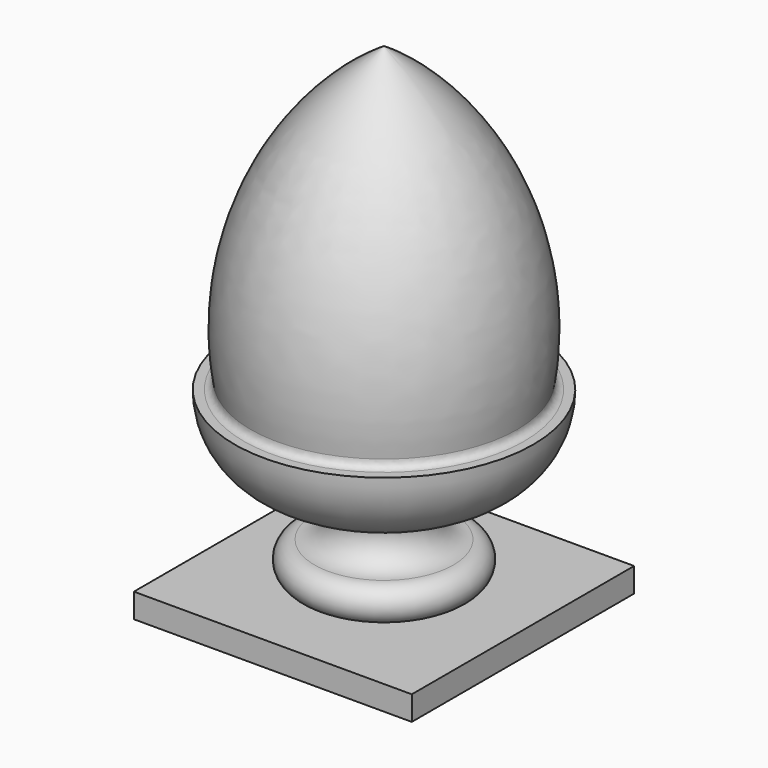
from build123d import *

# Parameters (mm, degrees)
F0_W     = 203.2
F0_H     = 203.2
F1_DEPTH = 17.78
F4_R     = 5.08


# Not quite as in the source:
# - a feature names something its author has since deleted; it is built from what else it names


with BuildPart() as f1:
    # F0 (on Top) → F1 (new body)
    with BuildSketch(Plane.XY):
        Rectangle(F0_W, F0_H)
    extrude(amount=F1_DEPTH)

    # F2 (on Front) → F3 (revolve)
    with BuildSketch(Plane.XZ):
        with BuildLine():
            Line((0, 360.68), (0, 17.78))
            Line((0, 17.78), (50.8, 17.78))
            ThreePointArc((50.8, 17.78), (63.5, 30.48), (50.8, 43.18))
            ThreePointArc((50.8, 43.18), (31.75, 62.23), (50.8, 81.28))
            ThreePointArc((50.8, 81.28), (92.1091781569, 98.3908218431), (109.22, 139.7))
            Line((109.22, 139.7), (96.52, 139.7))
            ThreePointArc((96.52, 139.7), (82.2548109307, 265.0383082226), (0, 360.68))
        make_face()
    revolve(axis=Axis((0, 0, 189.23), (0, 0, 1)))

    # F4
    f4_edges = [f1.edges().sort_by_distance(p)[0] for p in [
        (-96.52, 0, 139.7),
    ]]
    fillet(f4_edges, radius=F4_R)


solid = f1.part
